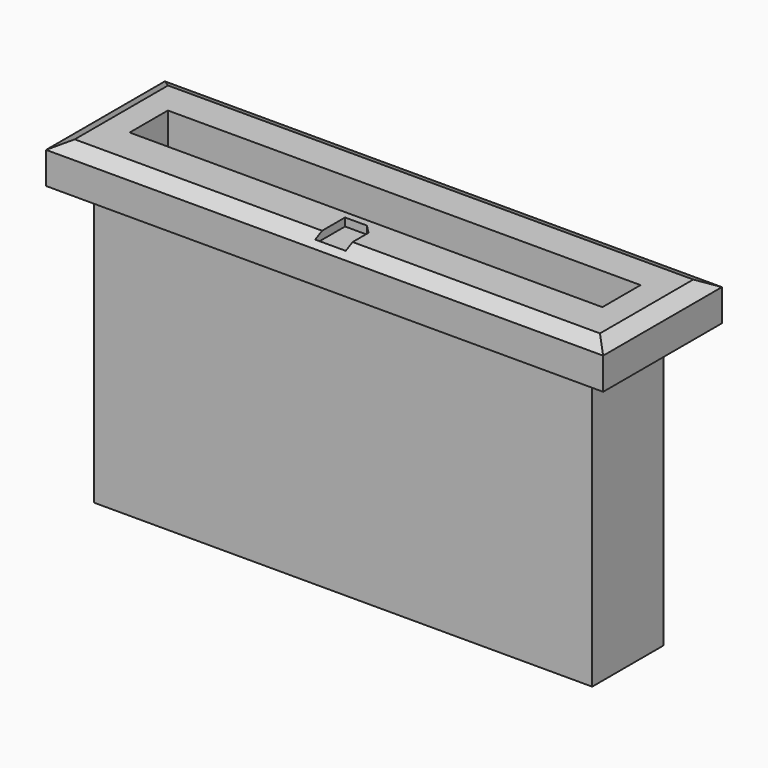
from build123d import *

# Parameters (mm, degrees)
F1_DEPTH    = 20
F2_START    = 18.5
F2_DEPTH    = 1.5
F3_START    = 17.5
F0_W        = 1.9191285201
F0_H        = 0.8
F3_DEPTH    = 2
F4_START    = 17.5
F0_H_2      = 0.9897637812
F4_DEPTH    = 2
F5_DEPTH    = 17.5
F6_DEPTH    = 18.5
F7_START    = 17.5
F0_W_2      = 35
F0_H_3      = 9.3263725303
F7_DEPTH    = 2.5
F8_T1_DEPTH = 40.1796577476
F8_T3_DEPTH = 14.5060302779


# Not quite as in the source:
# - a fillet or chamfer that OpenCascade refuses, or shapes differently, is made with other operations: its cross-section is extruded or revolved along the edge and cut away or added


with BuildPart() as f1:
    # F0 (on Top) → F1 (new body)
    with BuildSketch(Plane.XY):
        Polygon((-14.85, 2), (14.85, 2), (14.85, -1), (14.85, -2), (0.95956426, -2), (0.95956426, -2.8), (15.65, -2.8), (15.65, 2.8), (-15.65, 2.8), (-15.65, -2.8), (-0.95956426, -2.8), (-0.95956426, -2), (-14.85, -2), (-14.85, -1), align=None)
    extrude(amount=F1_DEPTH)

    # F0 (on Top) → F2 (join)
    with BuildSketch(Plane.XY.offset(F2_START)):
        Polygon((14.85, -2), (14.85, -1), (-14.85, -1), (-14.85, -2), (-0.95956426, -2), (-0.95956426, -1.4462094987), (0.4121778399, -1.4462094987), (0.95956426, -2), align=None)
    extrude(amount=F2_DEPTH)

    # F0 (on Top) → F3 (join)
    with BuildSketch(Plane.XY.offset(F3_START)):
        with Locations((0, -2.4)):
            Rectangle(F0_W, F0_H)
        Polygon((-0.95956426, -2), (0.95956426, -2), (0.4121778399, -1.4462094987), (-0.95956426, -1.4462094987), align=None)
    extrude(amount=F3_DEPTH)

    # F0 (on Top) → F4 (join)
    with BuildSketch(Plane.XY.offset(F4_START)):
        with Locations((0, -3.2948818906)):
            Rectangle(F0_W, F0_H_2)
    extrude(amount=F4_DEPTH)

    # F0 (on Top) → F5 (join)
    with BuildSketch(Plane.XY):
        with Locations((0, -2.4)):
            Rectangle(F0_W, F0_H)
    extrude(amount=F5_DEPTH)

    # F0 (on Top) → F6 (cut)
    with BuildSketch(Plane.XY):
        Polygon((-0.95956426, -2), (0.95956426, -2), (0.4121778399, -1.4462094987), (-0.95956426, -1.4462094987), align=None)
    extrude(amount=F6_DEPTH, mode=Mode.SUBTRACT)

    # F0 (on Top) → F7 (join)
    with BuildSketch(Plane.XY.offset(F7_START)):
        with Locations((0, 0.4131862652)):
            Rectangle(F0_W_2, F0_H_3)
        Polygon((15.65, -2.8), (0.95956426, -2.8), (0.95956426, -3.7897637812), (-0.95956426, -3.7897637812), (-0.95956426, -2.8), (-15.65, -2.8), (-15.65, 2.8), (15.65, 2.8), align=None, mode=Mode.SUBTRACT)
    extrude(amount=F7_DEPTH)

    # F8: chamfer of 0.5 x 1 on 4 edges, made by hand

    # F8_s2 → F8_t1 (cut)
    with BuildSketch(Plane.YZ.offset(-20.0898288738)):
        Polygon((4.0763725303, 20), (5.0763725303, 19.5), (5.0763725303, 20), align=None)
        Polygon((-3.25, 20), (-4.25, 19.5), (-4.25, 20), align=None)
    extrude(amount=F8_T1_DEPTH, mode=Mode.SUBTRACT)

    # F8_s4 → F8_t3 (cut)
    with BuildSketch(Plane.XZ.offset(-7.6662014041)):
        Polygon((-17.5, 19.5), (-16.5, 20), (-17.5, 20), align=None)
        Polygon((16.5, 20), (17.5, 19.5), (17.5, 20), align=None)
    extrude(amount=F8_T3_DEPTH, mode=Mode.SUBTRACT)


solid = f1.part
